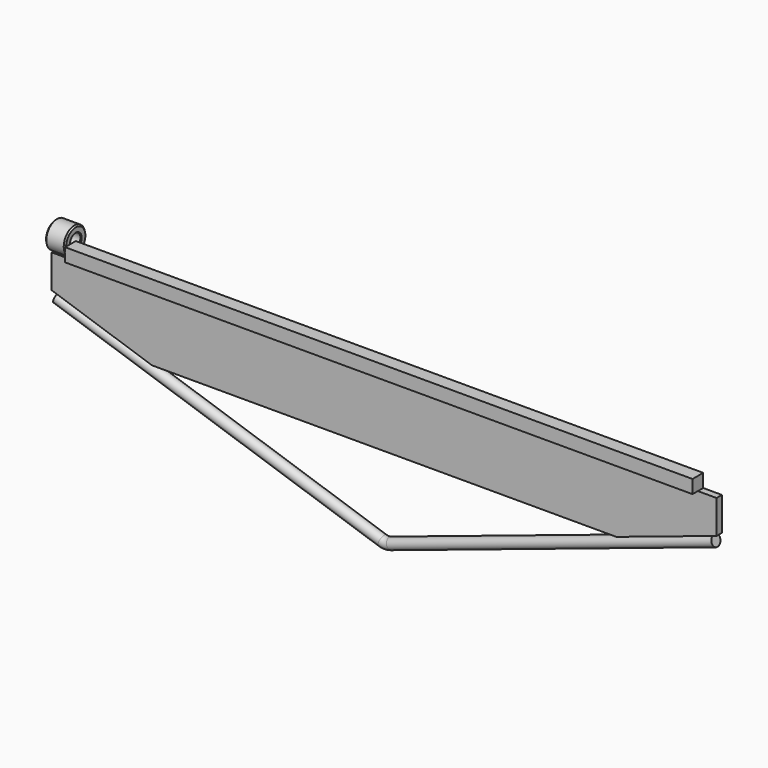
from build123d import *

# Parameters (mm, degrees)
F0_W      = 995
F0_H      = 120
F1_DEPTH  = 20
F2_W      = 28
F2_H      = 20
F3_DEPTH  = 25
F4_R      = 20
F4_R_2    = 10
F5_DEPTH  = 30
F6_SIZE   = 2
F7_SIZE   = 1
F9_DEPTH  = 10
F10_SIZE2 = 50
F10_SIZE  = 150
F14_R     = 8


# Not quite as in the source:
# - a pattern or mirror of a feature is missing from the dataset's text; its kind, count and spacing are read off the source's solid


with BuildPart() as f1:
    # F0 (on Front) → F1 (new body)
    with BuildSketch(Plane.XZ):
        Rectangle(F0_W, F0_H)
    extrude(amount=F1_DEPTH)

    # F2 (on Front) → F3 (cut)
    with BuildSketch(Plane.XZ):
        with Locations((-483.5, 50)):
            Rectangle(F2_W, F2_H)
    f3 = extrude(amount=F3_DEPTH, mode=Mode.SUBTRACT)

    # F3_copies: F3 across plane
    add(f3.mirror(Plane(origin=(0, 0, 0), x_dir=(0, 0, 1), z_dir=(1, 0, 0))), mode=Mode.SUBTRACT)

    # F8 (on face) → F9 (cut)
    with BuildSketch(Plane.XZ.offset(20)):
        Polygon((-497.5, 40), (-497.5, -60), (497.5, -60), (497.5, 40), (469.5, 40), (-469.5, 40), align=None)
    extrude(amount=-F9_DEPTH, mode=Mode.SUBTRACT)

    # F10
    f10_edges = [f1.edges().sort_by_distance(p)[0] for p in [
        (-497.5, -5, -60),
        (497.5, -5, -60),
    ]]
    f10_side = f1.faces().sort_by_distance((0, -5, -60))[0]
    chamfer(f10_edges, length=F10_SIZE, length2=F10_SIZE2, reference=f10_side)

    # F15: sweep along a path in F12
    with BuildLine(Plane.XZ.offset(5)) as f15_path:
        Line((-492.5, -19.5723608171), (-6.3245553203, -181.630842377))
        ThreePointArc((-6.3245553203, -181.630842377), (0, -182.657176416), (6.3245553203, -181.630842377))
        Line((6.3245553203, -181.630842377), (492.5, -19.5723608171))
    # F14 (on line) → F15 (sweep)
    with BuildSketch(Plane(origin=(-437.3782917549, 0, 145.7927639183), x_dir=(0, 1, 0), z_dir=(0.9486832981, 0, -0.316227766))):
        with Locations((-5, -174.3101465739)):
            Circle(F14_R)
    sweep(path=f15_path.line)


with BuildPart() as f5:
    # F4 (on face) → F5 (new body)
    with BuildSketch(Plane(origin=(-469.5, 0, 0), x_dir=(0, -1, 0), z_dir=(-1, 0, 0))):
        with Locations((0, 60)):
            Circle(F4_R)
        with Locations((0, 60)):
            Circle(F4_R_2, mode=Mode.SUBTRACT)
    extrude(amount=F5_DEPTH)

    # F6
    f6_edges = [f5.edges().sort_by_distance(p)[0] for p in [
        (-469.5, 20, 60),
        (-499.5, 20, 60),
    ]]
    chamfer(f6_edges, length=F6_SIZE)

    # F7
    f7_edges = [f5.edges().sort_by_distance(p)[0] for p in [
        (-469.5, 10, 60),
        (-499.5, 10, 60),
    ]]
    chamfer(f7_edges, length=F7_SIZE)


solid = Compound([f1.part, f5.part])
